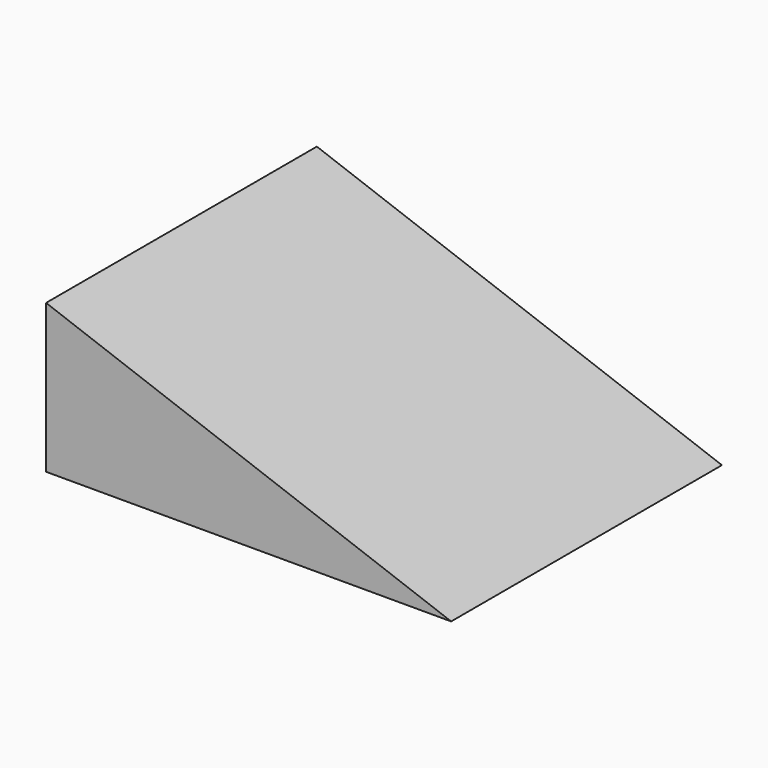
from build123d import *

# Parameters (mm, degrees)
F0_W     = 69.1770128906
F0_H     = 57.801194489
F1_DEPTH = 25.4
F3_DEPTH = 57.801194489


# Not quite as in the source:
# - the program builds the solid bodies; features that only make, move or delete a surface that nothing else refers to are left out


with BuildPart() as f1:
    # F0 (on Top) → F1 (new body)
    with BuildSketch(Plane.XY):
        with Locations((-5.8288183063, -0.5201026797)):
            Rectangle(F0_W, F0_H)
    extrude(amount=F1_DEPTH)

    # F2 (on face) → F3 (cut, through all)
    with BuildSketch(Plane.XZ.offset(29.4206999242)):
        Polygon((28.759688139, 25.4), (-40.4173247516, 25.4), (28.759688139, 0), align=None)
    extrude(amount=-F3_DEPTH, mode=Mode.SUBTRACT)


solid = f1.part
